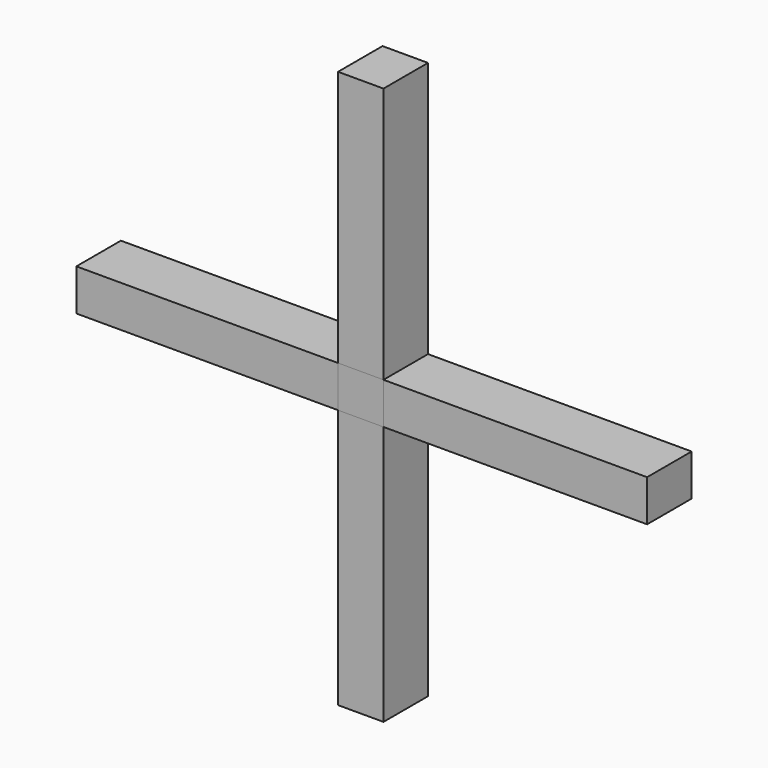
from build123d import *

# Parameters (mm, degrees)
F0_W     = 59.706710279
F0_H     = 9.4748688862
F1_DEPTH = 12.7
F0_W_2   = 10.3772366419
F0_H_2   = 58.5035607219
F0_W_3   = 60.1578941569
F0_H_3   = 59.2555301264
F2_DEPTH = 12.7


# Not quite as in the source:
# - a feature of the source that left no trace in its solid (it failed there, or was rolled back) is left out
# - the program builds the solid bodies; features that only make, move or delete a surface that nothing else refers to are left out


with BuildPart() as f1:
    # F0 (on Front) → F1 (new body)
    with BuildSketch(Plane.XZ):
        with Locations((-29.8533551395, -4.7374344431)):
            Rectangle(F0_W, F0_H)
    extrude(amount=F1_DEPTH)


with BuildPart() as f1b:
    # F0 (on Front) → F1, piece 2 (new body)
    with BuildSketch(Plane.XZ):
        with Locations((5.188618321, 29.2517803609)):
            Rectangle(F0_W_2, F0_H_2)
    extrude(amount=F1_DEPTH)


with BuildPart() as f1c:
    # F0 (on Front) → F1, piece 3 (new body)
    with BuildSketch(Plane.XZ):
        with Locations((40.4561837204, -4.7374344431)):
            Rectangle(F0_W_3, F0_H)
    extrude(amount=F1_DEPTH)


with BuildPart() as f1d:
    # F0 (on Front) → F1, piece 4 (new body)
    with BuildSketch(Plane.XZ):
        with Locations((5.188618321, -39.1026339494)):
            Rectangle(F0_W_2, F0_H_3)
    extrude(amount=F1_DEPTH)


with BuildPart() as f2:
    # F0 (on Front) → F2 (new body)
    with BuildSketch(Plane.XZ):
        with Locations((5.188618321, -4.7374344431)):
            Rectangle(F0_W_2, F0_H)
    extrude(amount=F2_DEPTH)


solid = Compound([f1.part, f1b.part, f1c.part, f1d.part, f2.part])
